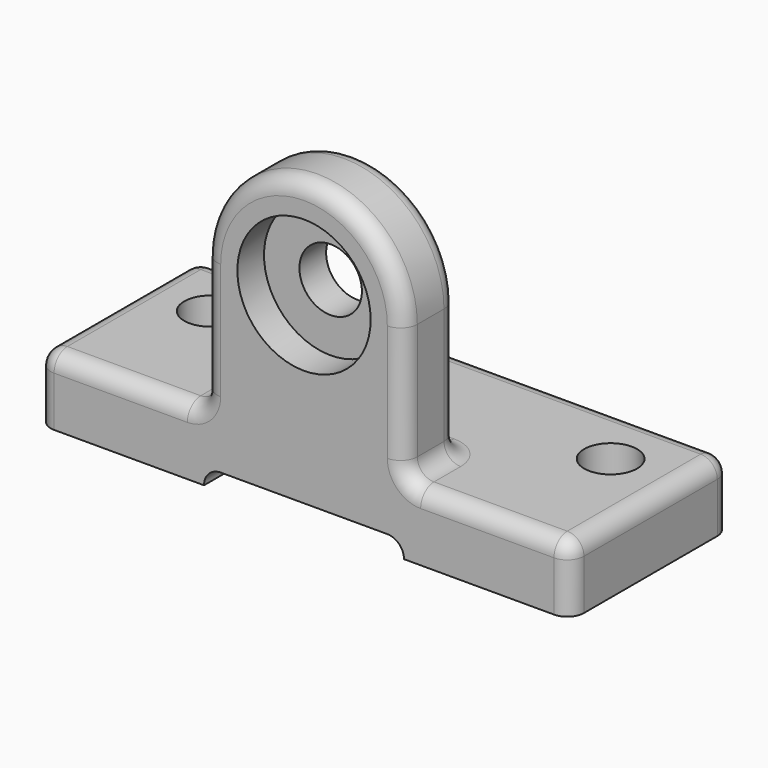
from build123d import *

# Parameters (mm, degrees)
F0_W           = 101.6
F0_H           = 38.1
F1_DEPTH       = 12.7
F3_DEPTH       = 12.7
F4_D           = 11.90625
F4_CBORE_D     = 25.4
F4_CBORE_DEPTH = 6.35
F5_W           = 38.1
F5_H           = 3.175
F6_DEPTH       = 38.101
F8_D           = 10.0838
F9_R           = 3.175
F10_R          = 3.175
F11_R          = 3.175
F12_R          = 3.17499
F13_R          = 3.175


# Not quite as in the source:
# - a fillet or chamfer is up to 0.001 mm smaller than in the source, because OpenCascade refuses the exact size
# - a length typed as a fraction of an inch, garbled in the dataset ("3 / 203.2 mm" for 3/8 in), is restored


with BuildPart() as f1:
    # F0 (on Top) → F1 (new body)
    with BuildSketch(Plane.XY):
        Rectangle(F0_W, F0_H)
    extrude(amount=F1_DEPTH)

    # F2 (on face) → F3 (join)
    with BuildSketch(Plane.XZ.offset(19.05)):
        with BuildLine():
            Line((-19.05, 38.1), (-19.05, 0))
            Line((-19.05, 0), (19.05, 0))
            Line((19.05, 0), (19.05, 38.1))
            ThreePointArc((19.05, 38.1), (0, 57.15), (-19.05, 38.1))
        make_face()
    extrude(amount=-F3_DEPTH)

    # F4 (through all)
    with Locations(Plane.XZ.offset(19.05)):
        with Locations((0, 38.1)):
            CounterBoreHole(F4_D / 2, F4_CBORE_D / 2, F4_CBORE_DEPTH)

    # F5 (on face) → F6 (cut, through all)
    with BuildSketch(Plane(origin=(0, 19.05, 0), x_dir=(-1, 0, 0), z_dir=(0, 1, 0))):
        with Locations((0, 1.5875)):
            Rectangle(F5_W, F5_H)
    extrude(amount=-F6_DEPTH, mode=Mode.SUBTRACT)

    # F8 (through all)
    with Locations(Plane.XY.offset(12.7)):
        with Locations((-38.1, 6.35), (38.1, 6.35)):
            Hole(F8_D / 2)

    # F9
    f9_edges = [f1.edges().sort_by_distance(p)[0] for p in [
        (-50.8, -19.05, 6.35),
    ]]
    fillet(f9_edges, radius=F9_R)

    # F10
    f10_edges = [f1.edges().sort_by_distance(p)[0] for p in [
        (-50.8, 19.05, 6.35),
        (50.8, -19.05, 6.35),
    ]]
    fillet(f10_edges, radius=F10_R)

    # F11
    f11_edges = [f1.edges().sort_by_distance(p)[0] for p in [
        (50.8, 19.05, 6.35),
    ]]
    fillet(f11_edges, radius=F11_R)

    # F12 (radius 3.175 in the source; OpenCascade refuses exactly that, so slightly less here)
    f12_edges = [f1.edges().sort_by_distance(p)[0] for p in [
        (-19.05, 0, 3.175),
        (19.05, 0, 3.175),
    ]]
    fillet(f12_edges, radius=F12_R)

    # F13
    f13_edges = [f1.edges().sort_by_distance(p)[0] for p in [
        (0, -19.05, 57.15),
        (19.05, -19.05, 25.4),
        (-19.05, -19.05, 25.4),
        (-33.3375, -19.05, 12.7),
        (33.3375, -19.05, 12.7),
        (49.870064, -18.120064, 12.7),
        (50.8, 0, 12.7),
        (0, 19.05, 12.7),
        (49.870064, 18.120064, 12.7),
        (-49.870064, 18.120064, 12.7),
        (-50.8, 0, 12.7),
        (-49.870064, -18.120064, 12.7),
        (19.05, -12.7, 12.7),
        (19.05, -6.35, 25.4),
        (0, -6.35, 57.15),
        (-19.05, -6.35, 25.4),
        (-19.05, -12.7, 12.7),
        (0, -6.35, 12.7),
    ]]
    fillet(f13_edges, radius=F13_R)


solid = f1.part
